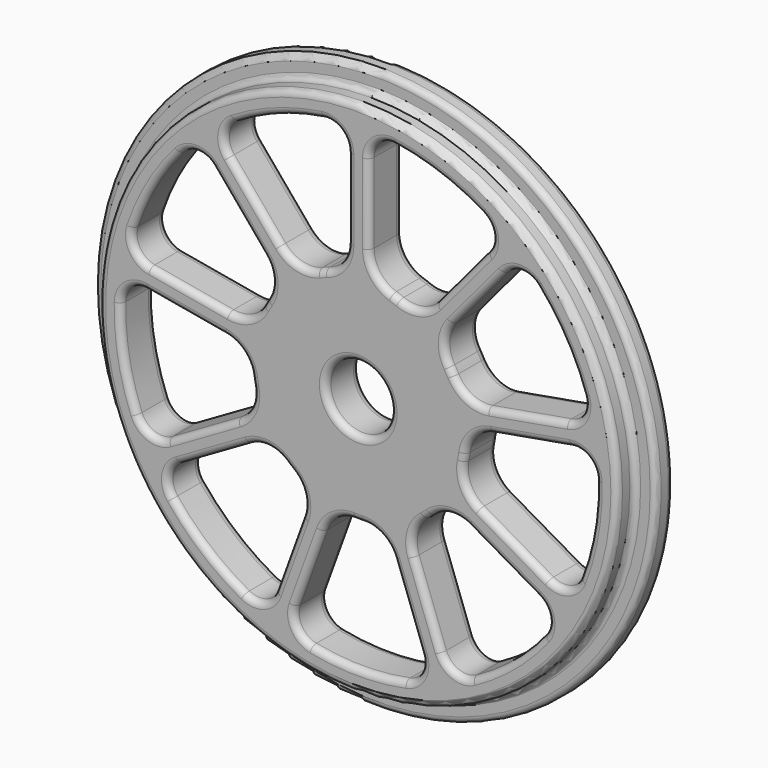
from build123d import *

# Parameters (mm, degrees)
F0_R     = 600
F0_R_2   = 75
F1_DEPTH = 100
F2_R     = 15
F3_R     = 650
F3_R_2   = 600
F3_R_3   = 75
F4_DEPTH = 50
F5_R     = 14
F6_R     = 15
F7_R     = 20


with BuildPart() as f1:
    # F0 (on Front) → F1 (new body)
    with BuildSketch(Plane.XZ):
        Circle(F0_R)
        with BuildLine():
            ThreePointArc((-429.6749542125, -343.3357448949), (-439.746414593, -302.8516185834), (-415.6135947386, -268.8221342607))
            Line((-415.6135947386, -268.8221342607), (-255.3035660704, -176.2670960553))
            ThreePointArc((-255.3035660704, -176.2670960553), (-209.9119989203, -166.6353357821), (-167.5412046695, -185.5530779532))
            ThreePointArc((-167.5412046695, -185.5530779532), (-160.6969024216, -191.5111107797), (-153.6408848886, -197.2168311546))
            ThreePointArc((-153.6408848886, -197.2168311546), (-127.6529345211, -235.6588863805), (-129.2562037962, -282.0333912504))
            Line((-129.2562037962, -282.0333912504), (-192.5675786612, -455.9799640867))
            ThreePointArc((-192.5675786612, -455.9799640867), (-221.8894584636, -485.655310121), (-263.5074306706, -482.7668526125))
            ThreePointArc((-263.5074306706, -482.7668526125), (-353.5331853276, -421.3244437154), (-429.6749542125, -343.3357448949))
        make_face(mode=Mode.SUBTRACT)
        with BuildLine():
            ThreePointArc((-549.8420738028, 13.1792972596), (-531.5345652794, 50.665747199), (-491.1740218465, 61.2215669775))
            Line((-491.1740218465, 61.2215669775), (-308.8761834364, 29.077539541))
            ThreePointArc((-308.8761834364, 29.077539541), (-267.9130494936, 7.2787590274), (-247.615228278, -34.4484937961))
            ThreePointArc((-247.615228278, -34.4484937961), (-246.2019382531, -43.4120444167), (-244.4642815926, -52.3184004479))
            ThreePointArc((-244.4642815926, -52.3184004479), (-249.2664334156, -98.4714557331), (-280.3035660704, -132.9658258661))
            Line((-280.3035660704, -132.9658258661), (-440.6135947386, -225.5208640715))
            ThreePointArc((-440.6135947386, -225.5208640715), (-482.150402567, -229.405756969), (-512.1749542125, -200.4415532705))
            ThreePointArc((-512.1749542125, -200.4415532705), (-541.6442641567, -95.5064977168), (-549.8420738028, 13.1792972596))
        make_face(mode=Mode.SUBTRACT)
        with BuildLine():
            ThreePointArc((-108.4581482409, -539.2001762612), (-142.1960292815, -514.6613462099), (-145.5829476219, -473.080971253))
            Line((-145.5829476219, -473.080971253), (-82.2715727569, -299.1343984167))
            ThreePointArc((-82.2715727569, -299.1343984167), (-53.6907911402, -262.5789050337), (-9.072789383, -249.8353147432))
            ThreePointArc((-9.072789383, -249.8353147432), (0, -250), (9.072789383, -249.8353147432))
            ThreePointArc((9.072789383, -249.8353147432), (53.6907911402, -262.5789050337), (82.2715727569, -299.1343984167))
            Line((82.2715727569, -299.1343984167), (145.5829476219, -473.080971253))
            ThreePointArc((145.5829476219, -473.080971253), (142.1960292815, -514.6613462099), (108.4581482409, -539.2001762612))
            ThreePointArc((108.4581482409, -539.2001762612), (0, -550), (-108.4581482409, -539.2001762612))
        make_face(mode=Mode.SUBTRACT)
        with BuildLine():
            ThreePointArc((263.5074306706, -482.7668526125), (221.8894584636, -485.655310121), (192.5675786612, -455.9799640867))
            Line((192.5675786612, -455.9799640867), (129.2562037962, -282.0333912504))
            ThreePointArc((129.2562037962, -282.0333912504), (127.6529345211, -235.6588863805), (153.6408848886, -197.2168311546))
            ThreePointArc((153.6408848886, -197.2168311546), (160.6969024216, -191.5111107797), (167.5412046695, -185.5530779532))
            ThreePointArc((167.5412046695, -185.5530779532), (209.9119989203, -166.6353357821), (255.3035660704, -176.2670960553))
            Line((255.3035660704, -176.2670960553), (415.6135947386, -268.8221342607))
            ThreePointArc((415.6135947386, -268.8221342607), (439.746414593, -302.8516185834), (429.6749542125, -343.3357448949))
            ThreePointArc((429.6749542125, -343.3357448949), (353.5331853276, -421.3244437154), (263.5074306706, -482.7668526125))
        make_face(mode=Mode.SUBTRACT)
        with BuildLine():
            ThreePointArc((512.1749542125, -200.4415532705), (482.150402567, -229.405756969), (440.6135947386, -225.5208640715))
            Line((440.6135947386, -225.5208640715), (280.3035660704, -132.9658258661))
            ThreePointArc((280.3035660704, -132.9658258661), (249.2664334156, -98.4714557331), (244.4642815926, -52.3184004479))
            ThreePointArc((244.4642815926, -52.3184004479), (246.2019382531, -43.4120444167), (247.615228278, -34.4484937961))
            ThreePointArc((247.615228278, -34.4484937961), (267.9130494936, 7.2787590274), (308.8761834364, 29.077539541))
            Line((308.8761834364, 29.077539541), (491.1740218465, 61.2215669775))
            ThreePointArc((491.1740218465, 61.2215669775), (531.5345652794, 50.665747199), (549.8420738028, 13.1792972596))
            ThreePointArc((549.8420738028, 13.1792972596), (541.6442641567, -95.5064977168), (512.1749542125, -200.4415532705))
        make_face(mode=Mode.SUBTRACT)
        with BuildLine():
            ThreePointArc((-217.9222017962, 220.8164712251), (-200.554606687, 177.7870415935), (-211.8273346385, 132.7749234605))
            ThreePointArc((-211.8273346385, 132.7749234605), (-216.5063509461, 125), (-220.9001240216, 117.0603912827))
            ThreePointArc((-220.9001240216, 117.0603912827), (-254.2453978272, 84.7918634401), (-300.1937745531, 78.3179271916))
            Line((-300.1937745531, 78.3179271916), (-482.4916129631, 110.4619546281))
            ThreePointArc((-482.4916129631, 110.4619546281), (-516.8078148044, 134.1852994299), (-521.1901244877, 175.6725765066))
            ThreePointArc((-521.1901244877, 175.6725765066), (-476.3139720814, 275), (-412.7319762468, 363.5275997547))
            ThreePointArc((-412.7319762468, 363.5275997547), (-374.6117855229, 380.47604678), (-336.9086653412, 362.6190166249))
            Line((-336.9086653412, 362.6190166249), (-217.9222017962, 220.8164712251))
        make_face(mode=Mode.SUBTRACT)
        with BuildLine():
            ThreePointArc((-286.3346431322, 469.587555353), (-188.1110788291, 516.8309414322), (-82.5, 543.7772981653))
            ThreePointArc((-82.5, 543.7772981653), (-42.403987974, 532.2573755524), (-25, 494.3429983321))
            Line((-25, 494.3429983321), (-25, 309.2329219213))
            ThreePointArc((-25, 309.2329219213), (-39.3544344953, 265.1067915152), (-76.9230769231, 237.871478401))
            ThreePointArc((-76.9230769231, 237.871478401), (-85.5050358314, 234.9231551965), (-93.9743433895, 231.6653249507))
            ThreePointArc((-93.9743433895, 231.6653249507), (-140.2601149725, 228.3801273531), (-179.6199796402, 252.9558517094))
            Line((-179.6199796402, 252.9558517094), (-298.6064431852, 394.7583971093))
            ThreePointArc((-298.6064431852, 394.7583971093), (-309.6451068158, 434.989562922), (-286.3346431322, 469.587555353))
        make_face(mode=Mode.SUBTRACT)
        Circle(F0_R_2, mode=Mode.SUBTRACT)
        with BuildLine():
            ThreePointArc((521.1901244877, 175.6725765066), (516.8078148044, 134.1852994299), (482.4916129631, 110.4619546281))
            Line((482.4916129631, 110.4619546281), (300.1937745531, 78.3179271916))
            ThreePointArc((300.1937745531, 78.3179271916), (254.2453978272, 84.7918634401), (220.9001240216, 117.0603912827))
            ThreePointArc((220.9001240216, 117.0603912827), (216.5063509461, 125), (211.8273346385, 132.7749234605))
            ThreePointArc((211.8273346385, 132.7749234605), (200.554606687, 177.7870415935), (217.9222017962, 220.8164712251))
            Line((217.9222017962, 220.8164712251), (336.9086653412, 362.6190166249))
            ThreePointArc((336.9086653412, 362.6190166249), (374.6117855229, 380.47604678), (412.7319762468, 363.5275997547))
            ThreePointArc((412.7319762468, 363.5275997547), (476.3139720814, 275), (521.1901244877, 175.6725765066))
        make_face(mode=Mode.SUBTRACT)
        with BuildLine():
            Line((25, 309.2329219213), (25, 494.3429983321))
            ThreePointArc((25, 494.3429983321), (42.403987974, 532.2573755524), (82.5, 543.7772981653))
            ThreePointArc((82.5, 543.7772981653), (188.1110788291, 516.8309414322), (286.3346431322, 469.587555353))
            ThreePointArc((286.3346431322, 469.587555353), (309.6451068158, 434.989562922), (298.6064431852, 394.7583971093))
            Line((298.6064431852, 394.7583971093), (179.6199796402, 252.9558517094))
            ThreePointArc((179.6199796402, 252.9558517094), (140.2601149725, 228.3801273531), (93.9743433895, 231.6653249507))
            ThreePointArc((93.9743433895, 231.6653249507), (85.5050358314, 234.9231551965), (76.9230769231, 237.871478401))
            ThreePointArc((76.9230769231, 237.871478401), (39.3544344953, 265.1067915152), (25, 309.2329219213))
        make_face(mode=Mode.SUBTRACT)
    extrude(amount=F1_DEPTH)

    # F2
    f2_edges = [f1.edges().sort_by_distance(p)[0] for p in [
        (-600, -100, 0),
        (-353.533185, -100, -421.324444),
        (-439.746415, -100, -302.851619),
        (-335.45858, -100, -222.544615),
        (-209.911999, -100, -166.635336),
        (-160.696902, -100, -191.511111),
        (-127.652935, -100, -235.658886),
        (-160.911891, -100, -369.006678),
        (-221.889458, -100, -485.65531),
        (-531.534565, -100, 50.665747),
        (-400.025103, -100, 45.149553),
        (-267.913049, -100, 7.278759),
        (-246.201938, -100, -43.412044),
        (-249.266433, -100, -98.471456),
        (-360.45858, -100, -179.243345),
        (-482.150403, -100, -229.405757),
        (-541.644264, -100, -95.506498),
        (0, -100, -550),
        (-142.196029, -100, -514.661346),
        (-113.92726, -100, -386.107685),
        (-53.690791, -100, -262.578905),
        (0, -100, -250),
        (53.690791, -100, -262.578905),
        (113.92726, -100, -386.107685),
        (142.196029, -100, -514.661346),
        (221.889458, -100, -485.65531),
        (160.911891, -100, -369.006678),
        (127.652935, -100, -235.658886),
        (160.696902, -100, -191.511111),
        (209.911999, -100, -166.635336),
        (335.45858, -100, -222.544615),
        (439.746415, -100, -302.851619),
        (353.533185, -100, -421.324444),
        (482.150403, -100, -229.405757),
        (360.45858, -100, -179.243345),
        (249.266433, -100, -98.471456),
        (246.201938, -100, -43.412044),
        (267.913049, -100, 7.278759),
        (400.025103, -100, 45.149553),
        (531.534565, -100, 50.665747),
        (541.644264, -100, -95.506498),
        (-277.415434, -100, 291.717744),
        (-200.554607, -100, 177.787042),
        (-216.506351, -100, 125),
        (-254.245398, -100, 84.791863),
        (-391.342694, -100, 94.389941),
        (-516.807815, -100, 134.185299),
        (-476.313972, -100, 275),
        (-374.611786, -100, 380.476047),
        (-309.645107, -100, 434.989563),
        (-188.111079, -100, 516.830941),
        (-42.403988, -100, 532.257376),
        (-25, -100, 401.78796),
        (-39.354434, -100, 265.106792),
        (-85.505036, -100, 234.923155),
        (-140.260115, -100, 228.380127),
        (-239.113211, -100, 323.857124),
        (-75, -100, 0),
        (476.313972, -100, 275),
        (516.807815, -100, 134.185299),
        (391.342694, -100, 94.389941),
        (254.245398, -100, 84.791863),
        (216.506351, -100, 125),
        (200.554607, -100, 177.787042),
        (277.415434, -100, 291.717744),
        (374.611786, -100, 380.476047),
        (25, -100, 401.78796),
        (42.403988, -100, 532.257376),
        (188.111079, -100, 516.830941),
        (309.645107, -100, 434.989563),
        (239.113211, -100, 323.857124),
        (140.260115, -100, 228.380127),
        (85.505036, -100, 234.923155),
        (39.354434, -100, 265.106792),
    ]]
    fillet(f2_edges, radius=F2_R)

    # F3 (on face) → F4 (join)
    with BuildSketch(Plane(origin=(0, 0, 0), x_dir=(-1, 0, 0), z_dir=(0, 1, 0))):
        Circle(F3_R)
        Circle(F3_R_2, mode=Mode.SUBTRACT)
        Circle(F3_R_2)
        with BuildLine():
            Line((-129.2562037962, -282.0333912504), (-192.5675786612, -455.9799640867))
            ThreePointArc((-192.5675786612, -455.9799640867), (-221.8894584636, -485.655310121), (-263.5074306706, -482.7668526125))
            ThreePointArc((-263.5074306706, -482.7668526125), (-353.5331853276, -421.3244437154), (-429.6749542125, -343.3357448949))
            ThreePointArc((-429.6749542125, -343.3357448949), (-439.746414593, -302.8516185834), (-415.6135947386, -268.8221342607))
            Line((-415.6135947386, -268.8221342607), (-255.3035660704, -176.2670960553))
            ThreePointArc((-255.3035660704, -176.2670960553), (-209.9119989203, -166.6353357821), (-167.5412046695, -185.5530779532))
            ThreePointArc((-167.5412046695, -185.5530779532), (-160.6969024216, -191.5111107797), (-153.6408848886, -197.2168311546))
            ThreePointArc((-153.6408848886, -197.2168311546), (-127.6529345211, -235.6588863805), (-129.2562037962, -282.0333912504))
        make_face(mode=Mode.SUBTRACT)
        with BuildLine():
            Line((-280.3035660704, -132.9658258661), (-440.6135947386, -225.5208640715))
            ThreePointArc((-440.6135947386, -225.5208640715), (-482.150402567, -229.405756969), (-512.1749542125, -200.4415532705))
            ThreePointArc((-512.1749542125, -200.4415532705), (-541.6442641567, -95.5064977168), (-549.8420738028, 13.1792972596))
            ThreePointArc((-549.8420738028, 13.1792972596), (-531.5345652794, 50.665747199), (-491.1740218465, 61.2215669775))
            Line((-491.1740218465, 61.2215669775), (-308.8761834364, 29.077539541))
            ThreePointArc((-308.8761834364, 29.077539541), (-267.9130494936, 7.2787590274), (-247.615228278, -34.4484937961))
            ThreePointArc((-247.615228278, -34.4484937961), (-246.2019382531, -43.4120444167), (-244.4642815926, -52.3184004479))
            ThreePointArc((-244.4642815926, -52.3184004479), (-249.2664334156, -98.4714557331), (-280.3035660704, -132.9658258661))
        make_face(mode=Mode.SUBTRACT)
        with BuildLine():
            ThreePointArc((145.5829476219, -473.080971253), (142.1960292815, -514.6613462099), (108.4581482409, -539.2001762612))
            ThreePointArc((108.4581482409, -539.2001762612), (0, -550), (-108.4581482409, -539.2001762612))
            ThreePointArc((-108.4581482409, -539.2001762612), (-142.1960292815, -514.6613462099), (-145.5829476219, -473.080971253))
            Line((-145.5829476219, -473.080971253), (-82.2715727569, -299.1343984167))
            ThreePointArc((-82.2715727569, -299.1343984167), (-53.6907911402, -262.5789050337), (-9.072789383, -249.8353147432))
            ThreePointArc((-9.072789383, -249.8353147432), (0, -250), (9.072789383, -249.8353147432))
            ThreePointArc((9.072789383, -249.8353147432), (53.6907911402, -262.5789050337), (82.2715727569, -299.1343984167))
            Line((82.2715727569, -299.1343984167), (145.5829476219, -473.080971253))
        make_face(mode=Mode.SUBTRACT)
        with BuildLine():
            ThreePointArc((415.6135947386, -268.8221342607), (439.746414593, -302.8516185834), (429.6749542125, -343.3357448949))
            ThreePointArc((429.6749542125, -343.3357448949), (353.5331853276, -421.3244437154), (263.5074306706, -482.7668526125))
            ThreePointArc((263.5074306706, -482.7668526125), (221.8894584636, -485.655310121), (192.5675786612, -455.9799640867))
            Line((192.5675786612, -455.9799640867), (129.2562037962, -282.0333912504))
            ThreePointArc((129.2562037962, -282.0333912504), (127.6529345211, -235.6588863805), (153.6408848886, -197.2168311546))
            ThreePointArc((153.6408848886, -197.2168311546), (160.6969024216, -191.5111107797), (167.5412046695, -185.5530779532))
            ThreePointArc((167.5412046695, -185.5530779532), (209.9119989203, -166.6353357821), (255.3035660704, -176.2670960553))
            Line((255.3035660704, -176.2670960553), (415.6135947386, -268.8221342607))
        make_face(mode=Mode.SUBTRACT)
        with BuildLine():
            Line((308.8761834364, 29.077539541), (491.1740218465, 61.2215669775))
            ThreePointArc((491.1740218465, 61.2215669775), (531.5345652794, 50.665747199), (549.8420738028, 13.1792972596))
            ThreePointArc((549.8420738028, 13.1792972596), (541.6442641567, -95.5064977168), (512.1749542125, -200.4415532705))
            ThreePointArc((512.1749542125, -200.4415532705), (482.150402567, -229.405756969), (440.6135947386, -225.5208640715))
            Line((440.6135947386, -225.5208640715), (280.3035660704, -132.9658258661))
            ThreePointArc((280.3035660704, -132.9658258661), (249.2664334156, -98.4714557331), (244.4642815926, -52.3184004479))
            ThreePointArc((244.4642815926, -52.3184004479), (246.2019382531, -43.4120444167), (247.615228278, -34.4484937961))
            ThreePointArc((247.615228278, -34.4484937961), (267.9130494936, 7.2787590274), (308.8761834364, 29.077539541))
        make_face(mode=Mode.SUBTRACT)
        with BuildLine():
            ThreePointArc((-482.4916129631, 110.4619546281), (-516.8078148044, 134.1852994299), (-521.1901244877, 175.6725765066))
            ThreePointArc((-521.1901244877, 175.6725765066), (-476.3139720814, 275), (-412.7319762468, 363.5275997547))
            ThreePointArc((-412.7319762468, 363.5275997547), (-374.6117855229, 380.47604678), (-336.9086653412, 362.6190166249))
            Line((-336.9086653412, 362.6190166249), (-217.9222017962, 220.8164712251))
            ThreePointArc((-217.9222017962, 220.8164712251), (-200.554606687, 177.7870415935), (-211.8273346385, 132.7749234605))
            ThreePointArc((-211.8273346385, 132.7749234605), (-216.5063509461, 125), (-220.9001240216, 117.0603912827))
            ThreePointArc((-220.9001240216, 117.0603912827), (-254.2453978272, 84.7918634401), (-300.1937745531, 78.3179271916))
            Line((-300.1937745531, 78.3179271916), (-482.4916129631, 110.4619546281))
        make_face(mode=Mode.SUBTRACT)
        with BuildLine():
            ThreePointArc((-82.5, 543.7772981653), (-42.403987974, 532.2573755524), (-25, 494.3429983321))
            Line((-25, 494.3429983321), (-25, 309.2329219213))
            ThreePointArc((-25, 309.2329219213), (-39.3544344953, 265.1067915152), (-76.9230769231, 237.871478401))
            ThreePointArc((-76.9230769231, 237.871478401), (-85.5050358314, 234.9231551965), (-93.9743433895, 231.6653249507))
            ThreePointArc((-93.9743433895, 231.6653249507), (-140.2601149725, 228.3801273531), (-179.6199796402, 252.9558517094))
            Line((-179.6199796402, 252.9558517094), (-298.6064431852, 394.7583971093))
            ThreePointArc((-298.6064431852, 394.7583971093), (-309.6451068158, 434.989562922), (-286.3346431322, 469.587555353))
            ThreePointArc((-286.3346431322, 469.587555353), (-188.1110788291, 516.8309414322), (-82.5, 543.7772981653))
        make_face(mode=Mode.SUBTRACT)
        Circle(F3_R_3, mode=Mode.SUBTRACT)
        with BuildLine():
            ThreePointArc((211.8273346385, 132.7749234605), (200.554606687, 177.7870415935), (217.9222017962, 220.8164712251))
            Line((217.9222017962, 220.8164712251), (336.9086653412, 362.6190166249))
            ThreePointArc((336.9086653412, 362.6190166249), (374.6117855229, 380.47604678), (412.7319762468, 363.5275997547))
            ThreePointArc((412.7319762468, 363.5275997547), (476.3139720814, 275), (521.1901244877, 175.6725765066))
            ThreePointArc((521.1901244877, 175.6725765066), (516.8078148044, 134.1852994299), (482.4916129631, 110.4619546281))
            Line((482.4916129631, 110.4619546281), (300.1937745531, 78.3179271916))
            ThreePointArc((300.1937745531, 78.3179271916), (254.2453978272, 84.7918634401), (220.9001240216, 117.0603912827))
            ThreePointArc((220.9001240216, 117.0603912827), (216.5063509461, 125), (211.8273346385, 132.7749234605))
        make_face(mode=Mode.SUBTRACT)
        with BuildLine():
            ThreePointArc((82.5, 543.7772981653), (188.1110788291, 516.8309414322), (286.3346431322, 469.587555353))
            ThreePointArc((286.3346431322, 469.587555353), (309.6451068158, 434.989562922), (298.6064431852, 394.7583971093))
            Line((298.6064431852, 394.7583971093), (179.6199796402, 252.9558517094))
            ThreePointArc((179.6199796402, 252.9558517094), (140.2601149725, 228.3801273531), (93.9743433895, 231.6653249507))
            ThreePointArc((93.9743433895, 231.6653249507), (85.5050358314, 234.9231551965), (76.9230769231, 237.871478401))
            ThreePointArc((76.9230769231, 237.871478401), (39.3544344953, 265.1067915152), (25, 309.2329219213))
            Line((25, 309.2329219213), (25, 494.3429983321))
            ThreePointArc((25, 494.3429983321), (42.403987974, 532.2573755524), (82.5, 543.7772981653))
        make_face(mode=Mode.SUBTRACT)
    extrude(amount=-F4_DEPTH)

    # F5
    f5_edges = [f1.edges().sort_by_distance(p)[0] for p in [
        (650, -50, 0),
        (-600, -50, 0),
    ]]
    fillet(f5_edges, radius=F5_R)

    # F6
    f6_edges = [f1.edges().sort_by_distance(p)[0] for p in [
        (650, 0, 0),
    ]]
    fillet(f6_edges, radius=F6_R)

    # F7
    f7_edges = [f1.edges().sort_by_distance(p)[0] for p in [
        (635, 0, 0),
        (-353.533185, 0, -421.324444),
        (-439.746415, 0, -302.851619),
        (-335.45858, 0, -222.544615),
        (-209.911999, 0, -166.635336),
        (-160.696902, 0, -191.511111),
        (-127.652935, 0, -235.658886),
        (-160.911891, 0, -369.006678),
        (-221.889458, 0, -485.65531),
        (-531.534565, 0, 50.665747),
        (-400.025103, 0, 45.149553),
        (-267.913049, 0, 7.278759),
        (-246.201938, 0, -43.412044),
        (-249.266433, 0, -98.471456),
        (-360.45858, 0, -179.243345),
        (-482.150403, 0, -229.405757),
        (-541.644264, 0, -95.506498),
        (0, 0, -550),
        (-142.196029, 0, -514.661346),
        (-113.92726, 0, -386.107685),
        (-53.690791, 0, -262.578905),
        (0, 0, -250),
        (53.690791, 0, -262.578905),
        (113.92726, 0, -386.107685),
        (142.196029, 0, -514.661346),
        (221.889458, 0, -485.65531),
        (160.911891, 0, -369.006678),
        (127.652935, 0, -235.658886),
        (160.696902, 0, -191.511111),
        (209.911999, 0, -166.635336),
        (335.45858, 0, -222.544615),
        (439.746415, 0, -302.851619),
        (353.533185, 0, -421.324444),
        (482.150403, 0, -229.405757),
        (360.45858, 0, -179.243345),
        (249.266433, 0, -98.471456),
        (246.201938, 0, -43.412044),
        (267.913049, 0, 7.278759),
        (400.025103, 0, 45.149553),
        (531.534565, 0, 50.665747),
        (541.644264, 0, -95.506498),
        (-277.415434, 0, 291.717744),
        (-200.554607, 0, 177.787042),
        (-216.506351, 0, 125),
        (-254.245398, 0, 84.791863),
        (-391.342694, 0, 94.389941),
        (-516.807815, 0, 134.185299),
        (-476.313972, 0, 275),
        (-374.611786, 0, 380.476047),
        (-309.645107, 0, 434.989563),
        (-188.111079, 0, 516.830941),
        (-42.403988, 0, 532.257376),
        (-25, 0, 401.78796),
        (-39.354434, 0, 265.106792),
        (-85.505036, 0, 234.923155),
        (-140.260115, 0, 228.380127),
        (-239.113211, 0, 323.857124),
        (-75, 0, 0),
        (476.313972, 0, 275),
        (516.807815, 0, 134.185299),
        (391.342694, 0, 94.389941),
        (254.245398, 0, 84.791863),
        (216.506351, 0, 125),
        (200.554607, 0, 177.787042),
        (277.415434, 0, 291.717744),
        (374.611786, 0, 380.476047),
        (25, 0, 401.78796),
        (42.403988, 0, 532.257376),
        (188.111079, 0, 516.830941),
        (309.645107, 0, 434.989563),
        (239.113211, 0, 323.857124),
        (140.260115, 0, 228.380127),
        (85.505036, 0, 234.923155),
        (39.354434, 0, 265.106792),
    ]]
    fillet(f7_edges, radius=F7_R)


solid = f1.part
